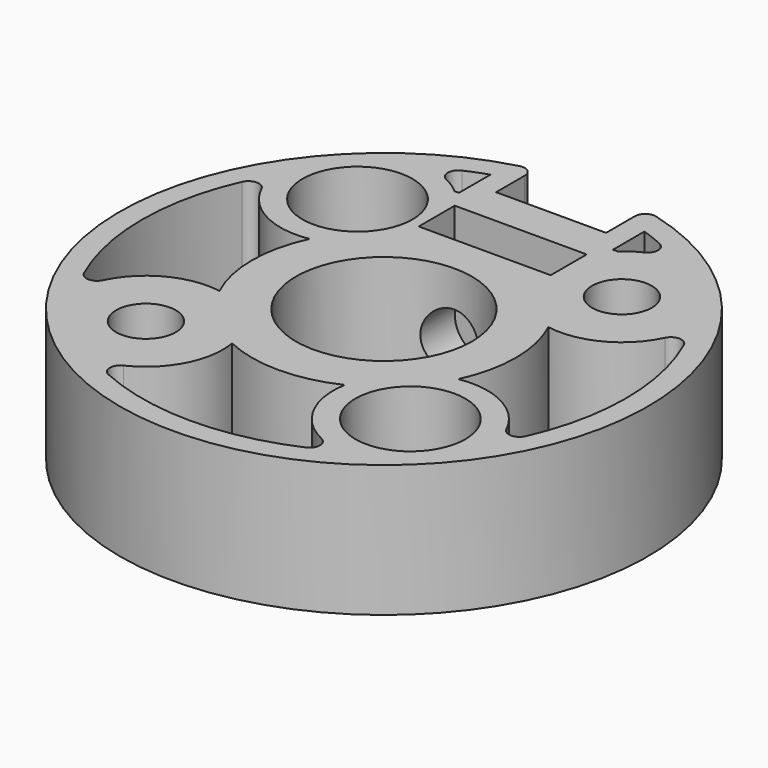
from build123d import *

# Parameters (mm, degrees)
F0_R             = 2.15265
F0_R_2           = 6.35
F1_DEPTH         = 9.525
F2_R             = 2.15265
F3_REACH         = 40.2208636501
F6_R             = 3.96875
F7_DEPTH         = 6.35
F8_R             = 3.96875
F9_DEPTH         = 6.35
F11_DEPTH        = 9.525
F11_COPIES_COUNT = 3
F11_COPIES_ANGLE = 180
F12_R            = 2.15265
F13_REACH        = 40.2208636501
F15_DEPTH        = 9.525
F16_R            = 0.762


# Not quite as in the source:
# - a pattern or mirror of a feature is missing from the dataset's text; its kind, count and spacing are read off the source's solid


with BuildPart() as f1:
    # F0 (on Top) → F1 (new body)
    with BuildSketch(Plane.XY):
        with BuildLine():
            Line((3.96875, 15.08125), (0, 15.08125))
            Line((0, 15.08125), (-3.96875, 15.08125))
            Line((-3.96875, 15.08125), (-3.96875, 18.6320026685))
            ThreePointArc((-3.96875, 18.6320026685), (0, -19.05), (3.96875, 18.6320026685))
            Line((3.96875, 18.6320026685), (3.96875, 15.08125))
        make_face()
        with Locations((-9.5415221286, -9.5415221286)):
            Circle(F0_R, mode=Mode.SUBTRACT)
        with Locations((9.5415221286, -9.5415221286)):
            Circle(F0_R, mode=Mode.SUBTRACT)
        Circle(F0_R_2, mode=Mode.SUBTRACT)
        with Locations((-9.5415221286, 9.5415221286)):
            Circle(F0_R, mode=Mode.SUBTRACT)
        Polygon((-4.7625, 12.341225), (0, 12.341225), (4.7625, 12.341225), (4.7625, 9.090025), (-4.7625, 9.090025), align=None, mode=Mode.SUBTRACT)
        with Locations((9.5415221286, 9.5415221286)):
            Circle(F0_R, mode=Mode.SUBTRACT)
    extrude(amount=F1_DEPTH)

    f3_end = f1.faces().sort_by_distance((-6.35, 0, 4.7625))[0]
    # F2 (on face) → F3 (cut, up to a face of the model that its end follows)
    with BuildSketch(Plane(origin=(0, 15.08125, 0), x_dir=(-1, 0, 0), z_dir=(0, 1, 0))):
        with Locations((0, 4.7625)):
            Circle(F2_R)
    f3_long = extrude(amount=-F3_REACH, mode=Mode.PRIVATE)
    add(split(f3_long, bisect_by=f3_end, keep=Keep.ALL, mode=Mode.PRIVATE).solids().sort_by_distance((0, 15.08125, 4.7625))[0], mode=Mode.SUBTRACT)

    # F6 (on face) → F7 (cut, through all)
    with BuildSketch(Plane.XY.offset(9.525)):
        with Locations((-9.5415221286, 9.5415221286)):
            Circle(F6_R)
        with Locations((9.5415221286, -9.5415221286)):
            Circle(F6_R)
    extrude(amount=-F7_DEPTH, mode=Mode.SUBTRACT)

    # F8 (on face) → F9 (cut, through all)
    with BuildSketch(Plane(origin=(0, 0, 0), x_dir=(1, 0, 0), z_dir=(0, 0, -1))):
        with Locations((9.5415221286, -9.5415221286)):
            Circle(F8_R)
        with Locations((-9.5415221286, 9.5415221286)):
            Circle(F8_R)
    extrude(amount=-F9_DEPTH, mode=Mode.SUBTRACT)

    # F10 (on face) → F11 (cut, through all)
    with BuildSketch(Plane.XY.offset(9.525)):
        with BuildLine():
            ThreePointArc((-8.6149297856, 4.0630788559), (-12.8558230168, 5.0820015619), (-15.0544327217, 8.8488960712))
            ThreePointArc((-15.0544327217, 8.8488960712), (-17.4625, 0), (-15.0544327217, -8.8488960712))
            ThreePointArc((-15.0544327217, -8.8488960712), (-12.8558230168, -5.0820015619), (-8.6149297856, -4.0630788559))
            ThreePointArc((-8.6149297856, -4.0630788559), (-9.525, 0), (-8.6149297856, 4.0630788559))
        make_face()
    f11 = extrude(amount=-F11_DEPTH, mode=Mode.SUBTRACT)

    # F11_copies: F11 ×3 about axis
    f11_copies_axis = Axis((0, 0, 0), (0, 0, 1))
    for i in range(1, F11_COPIES_COUNT):
        add(f11.rotate(f11_copies_axis, i * F11_COPIES_ANGLE / (F11_COPIES_COUNT - 1)), mode=Mode.SUBTRACT)

    f13_end = f1.faces().sort_by_distance((-6.35, 0, 4.7625))[0]
    # F12 (on face) → F13 (cut, up to a face of the model that its end follows)
    with BuildSketch(Plane(origin=(0, 15.08125, 0), x_dir=(-1, 0, 0), z_dir=(0, 1, 0))):
        with Locations((0, 4.7625)):
            Circle(F12_R)
    f13_long = extrude(amount=-F13_REACH, mode=Mode.PRIVATE)
    add(split(f13_long, bisect_by=f13_end, keep=Keep.TOP, mode=Mode.PRIVATE), mode=Mode.SUBTRACT)

    # F14 (on face) → F15 (cut, through all)
    with BuildSketch(Plane.XY.offset(9.525)):
        with BuildLine():
            ThreePointArc((-8.8488960712, 15.0544327217), (-7.2614037918, 14.6083726724), (-5.8747371797, 13.7160403285))
            Line((-5.8747371797, 13.7160403285), (-5.55625, 13.7160403285))
            Line((-5.55625, 13.7160403285), (-5.55625, 16.5549688066))
            ThreePointArc((-5.55625, 16.5549688066), (-7.2415440666, 15.8902154102), (-8.8488960712, 15.0544327217))
        make_face()
        with BuildLine():
            ThreePointArc((8.8488960712, 15.0544327217), (7.2415440666, 15.8902154102), (5.55625, 16.5549688066))
            Line((5.55625, 16.5549688066), (5.55625, 13.7160403285))
            Line((5.55625, 13.7160403285), (5.8747371797, 13.7160403285))
            ThreePointArc((5.8747371797, 13.7160403285), (7.2614037918, 14.6083726724), (8.8488960712, 15.0544327217))
        make_face()
    extrude(amount=-F15_DEPTH, mode=Mode.SUBTRACT)

    # F16
    f16_edges = [f1.edges().sort_by_distance(p)[0] for p in [
        (-15.054433, -8.848896, 4.7625),
        (-15.054433, 8.848896, 4.7625),
        (8.848896, 15.054433, 4.7625),
        (3.96875, 18.632003, 4.7625),
        (-3.96875, 18.632003, 4.7625),
        (-8.848896, 15.054433, 4.7625),
        (-8.848896, -15.054433, 4.7625),
        (8.848896, -15.054433, 4.7625),
        (15.054433, -8.848896, 4.7625),
        (15.054433, 8.848896, 4.7625),
    ]]
    fillet(f16_edges, radius=F16_R)


solid = f1.part
